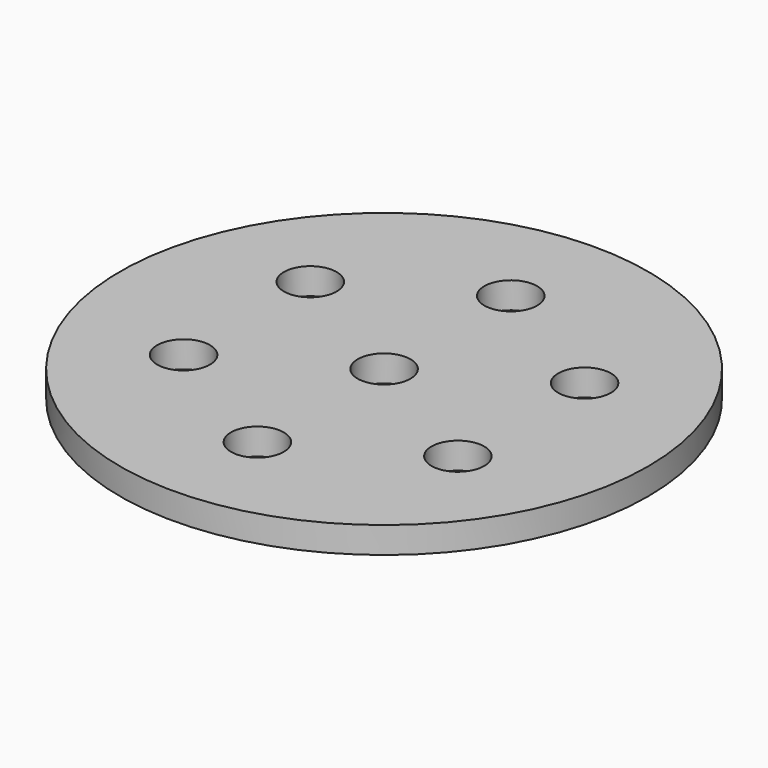
from build123d import *

# Parameters (mm, degrees)
F0_R            = 50
F0_R_2          = 5
F1_DEPTH        = 5
F2_R            = 5
F3_DEPTH        = 25
F3_COPIES_COUNT = 6


# Not quite as in the source:
# - a pattern or mirror of a feature is missing from the dataset's text; its kind, count and spacing are read off the source's solid


with BuildPart() as f1:
    # F0 (on Top) → F1 (new body)
    with BuildSketch(Plane.XY):
        Circle(F0_R)
        Circle(F0_R_2, mode=Mode.SUBTRACT)
    extrude(amount=F1_DEPTH)

    # F2 (on face) → F3 (cut)
    with BuildSketch(Plane.XY.offset(5)):
        with Locations((0, 30)):
            Circle(F2_R)
    f3 = extrude(amount=-F3_DEPTH, mode=Mode.SUBTRACT)

    # F3_copies: F3 ×6 about axis
    f3_copies_axis = Axis((0, 0, 0), (0, 0, 1))
    for i in range(1, F3_COPIES_COUNT):
        add(f3.rotate(f3_copies_axis, i * 360 / F3_COPIES_COUNT), mode=Mode.SUBTRACT)


solid = f1.part
